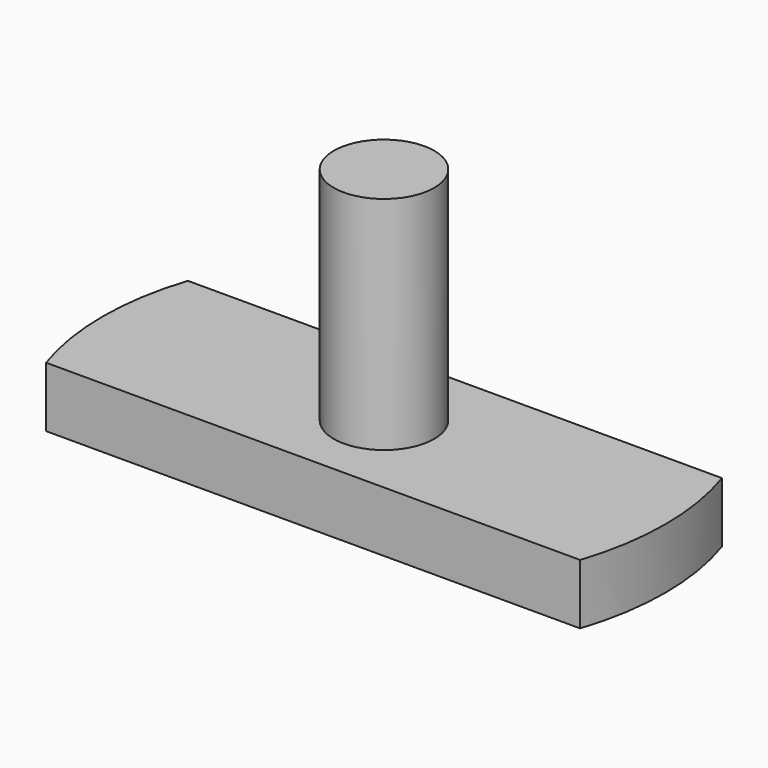
from build123d import *

# Parameters (mm, degrees)
F1_DEPTH       = 3
F2_D           = 0.34
F2_DEPTH       = 2
F2_CSINK_D     = 0.63
F2_CSINK_ANGLE = 90
F2_TIP         = 0.1021463052
F5_R           = 2.5
F6_DEPTH       = 14


# Not quite as in the source:
# - the program builds the solid bodies; features that only make, move or delete a surface that nothing else refers to are left out


with BuildPart() as f1:
    # F0 (on Top) → F1 (new body)
    with BuildSketch(Plane.XY):
        with BuildLine():
            Line((13.2871780876, 4.4103172753), (-13.2871780876, 4.4103172753))
            ThreePointArc((-13.2871780876, 4.4103172753), (-14, 0), (-13.2871780876, -4.4103172753))
            Line((-13.2871780876, -4.4103172753), (13.2871780876, -4.4103172753))
            ThreePointArc((13.2871780876, -4.4103172753), (14, 0), (13.2871780876, 4.4103172753))
        make_face()
    extrude(amount=F1_DEPTH)

    # F2
    with Locations(Plane(origin=(0, 0, 0), x_dir=(1, 0, 0), z_dir=(0, 0, -1))):
        with Locations((-10, 0), (10, 0)):
            CounterSinkHole(F2_D / 2, F2_CSINK_D / 2, depth=F2_DEPTH, counter_sink_angle=F2_CSINK_ANGLE)
            with Locations((0, 0, -(F2_DEPTH + F2_TIP / 2))):  # 118° drill point
                Cone(0, F2_D / 2, F2_TIP, mode=Mode.SUBTRACT)

    # F5 (on Top) → F6 (join)
    with BuildSketch(Plane.XY):
        Circle(F5_R)
    extrude(amount=F6_DEPTH)


solid = f1.part
